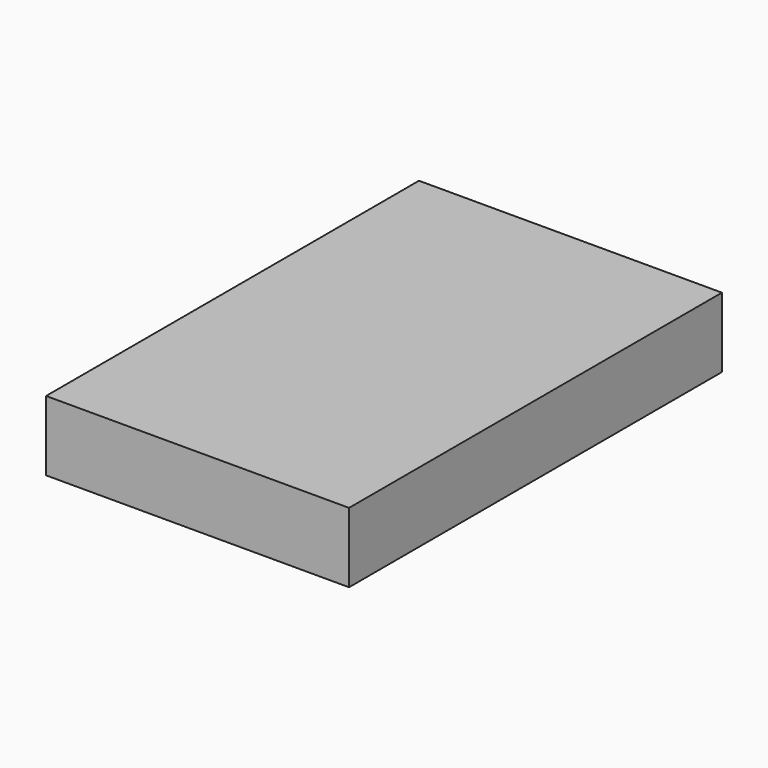
from build123d import *

# Parameters (mm, degrees)
F2_DEPTH = 63.5


# Not quite as in the source:
# - a feature of the source that left no trace in its solid (it failed there, or was rolled back) is left out


with BuildPart() as f2:
    # F0 (on Front) → F2 (new body, symmetric)
    with BuildSketch(Plane.XZ):
        Polygon((-41.275, -9.525), (41.275, -9.525), (41.275, 9.525), (22.225, 9.525), (-41.275, 9.525), align=None)
    extrude(amount=F2_DEPTH, both=True)


solid = f2.part
